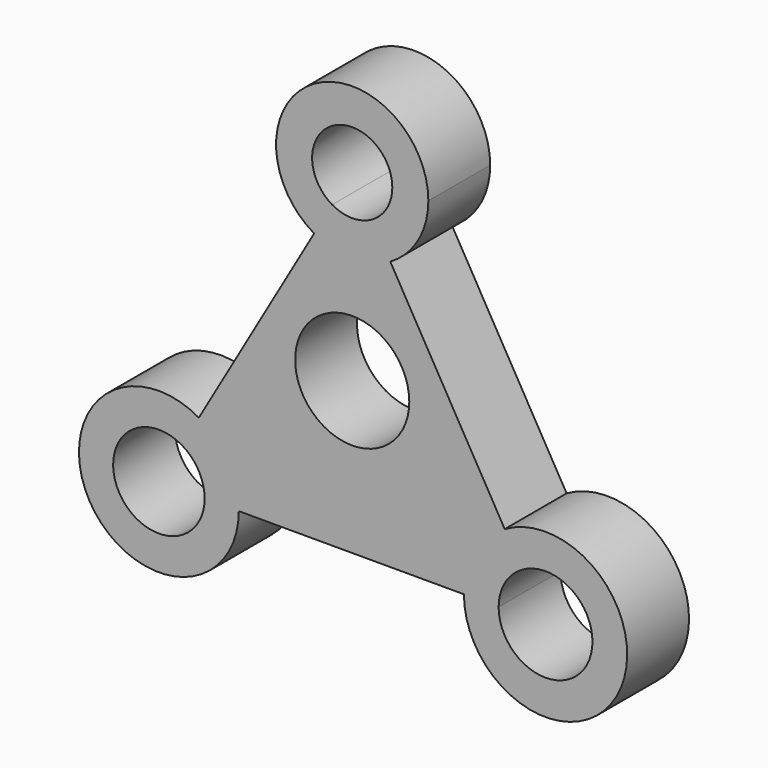
from build123d import *

# Parameters (mm, degrees)
F0_R     = 18.7435509256
F1_DEPTH = 25.4


with BuildPart() as f1:
    # F0 (on Front) → F1 (new body)
    with BuildSketch(Plane.XZ):
        with BuildLine():
            Line((-12.5020157932, 38.4971815486), (-6.5838834434, 48.7476874643))
            ThreePointArc((-6.5838834434, 48.7476874643), (-6.5838834434, 71.5549287346), (13.1677668869, 60.1513080994))
            ThreePointArc((13.1677668869, 60.1513080994), (11.4036206351, 53.567424656), (6.5838834434, 48.7476874643))
            Line((6.5838834434, 48.7476874643), (12.5020157932, 38.4971815486))
            ThreePointArc((12.5020157932, 38.4971815486), (21.6541265509, 47.6492923062), (25.0040315864, 60.1513080994))
            ThreePointArc((25.0040315864, 60.1513080994), (-12.5020157932, 81.8054346503), (-12.5020157932, 38.4971815486))
        make_face()
        with BuildLine():
            ThreePointArc((6.5838834434, 48.7476874643), (0, 46.9835412126), (-6.5838834434, 48.7476874643))
            Line((-6.5838834434, 48.7476874643), (-12.5020157932, 38.4971815486))
            ThreePointArc((-12.5020157932, 38.4971815486), (0, 35.147276513), (12.5020157932, 38.4971815486))
            Line((12.5020157932, 38.4971815486), (6.5838834434, 48.7476874643))
        make_face()
        with BuildLine():
            ThreePointArc((12.5020157932, 38.4971815486), (0, 35.147276513), (-12.5020157932, 38.4971815486))
            Line((-12.5020157932, 38.4971815486), (-50.3756712224, -27.1019139232))
            ThreePointArc((-50.3756712224, -27.1019139232), (-40.767995742, -36.7095894036), (-37.2513424448, -49.8339181812))
            Line((-37.2513424448, -49.8339181812), (36.6895705679, -49.8339181812))
            ThreePointArc((36.6895705679, -49.8339181812), (40.2814870254, -36.4287034651), (50.094785284, -26.6154052066))
            Line((50.094785284, -26.6154052066), (12.5020157932, 38.4971815486))
        make_face()
        Circle(F0_R, mode=Mode.SUBTRACT)
        with BuildLine():
            Line((55.796700688, -36.491412387), (50.094785284, -26.6154052066))
            ThreePointArc((50.094785284, -26.6154052066), (40.2814870254, -36.4287034651), (36.6895705679, -49.8339181812))
            Line((36.6895705679, -49.8339181812), (48.0934013761, -49.8339181812))
            ThreePointArc((48.0934013761, -49.8339181812), (50.1574942058, -42.1306188692), (55.796700688, -36.491412387))
        make_face()
        with BuildLine():
            ThreePointArc((90.3104294321, -49.8339181812), (76.905214716, -26.6154052066), (50.094785284, -26.6154052066))
            Line((50.094785284, -26.6154052066), (55.796700688, -36.491412387))
            ThreePointArc((55.796700688, -36.491412387), (71.203299312, -36.491412387), (78.9065986239, -49.8339181812))
            ThreePointArc((78.9065986239, -49.8339181812), (63.5, -65.2405168051), (48.0934013761, -49.8339181812))
            Line((48.0934013761, -49.8339181812), (36.6895705679, -49.8339181812))
            ThreePointArc((36.6895705679, -49.8339181812), (63.5, -76.6443476133), (90.3104294321, -49.8339181812))
        make_face()
        with BuildLine():
            ThreePointArc((-37.2513424448, -49.8339181812), (-40.767995742, -36.7095894036), (-50.3756712224, -27.1019139232))
            Line((-50.3756712224, -27.1019139232), (-55.9869244457, -36.8208896001))
            ThreePointArc((-55.9869244457, -36.8208896001), (-50.4869714189, -42.3208426269), (-48.4738488914, -49.8339181812))
            Line((-48.4738488914, -49.8339181812), (-37.2513424448, -49.8339181812))
        make_face()
        with BuildLine():
            Line((-55.9869244457, -36.8208896001), (-50.3756712224, -27.1019139232))
            ThreePointArc((-50.3756712224, -27.1019139232), (-86.232004258, -62.9582469588), (-37.2513424448, -49.8339181812))
            Line((-37.2513424448, -49.8339181812), (-48.4738488914, -49.8339181812))
            ThreePointArc((-48.4738488914, -49.8339181812), (-76.5130285811, -57.3469937355), (-55.9869244457, -36.8208896001))
        make_face()
    extrude(amount=F1_DEPTH)


solid = f1.part
